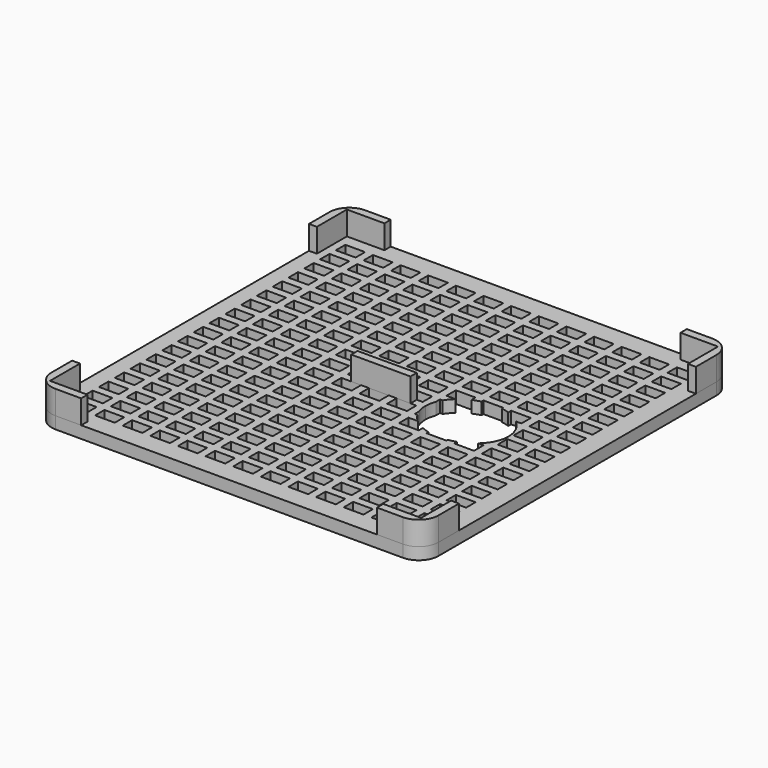
from build123d import *

# Parameters (mm, degrees)
F0_W     = 5
F0_H     = 3
F1_DEPTH = 3.048
F3_DEPTH = 4
F4_W     = 15
F4_H     = 2
F4_W_2   = 2
F4_W_3   = 9.6
F4_H_2   = 9.5
F4_W_4   = 9.5
F5_DEPTH = 6
F6_R     = 5


with BuildPart() as f1:
    # F0 (on Top) → F1 (new body)
    with BuildSketch(Plane.XY):
        Polygon((-42.5, 49), (-49, 49), (-49, 42.5), (-45, 42.5), (-45, 44), (-42.5, 44), align=None)
        Polygon((49, 49), (-42.5, 49), (-42.5, 44), (-40, 44), (-40, 41), (-45, 41), (-45, 42.5), (-49, 42.5), (-49, -49), (49, -49), align=None)
        with Locations((-42.5, -42.5)):
            Rectangle(F0_W, F0_H, mode=Mode.SUBTRACT)
        with Locations((-42.5, -37.5)):
            Rectangle(F0_W, F0_H, mode=Mode.SUBTRACT)
        with Locations((-35.5, -42.5)):
            Rectangle(F0_W, F0_H, mode=Mode.SUBTRACT)
        with Locations((-35.5, -37.5)):
            Rectangle(F0_W, F0_H, mode=Mode.SUBTRACT)
        with Locations((-28.5, -42.5)):
            Rectangle(F0_W, F0_H, mode=Mode.SUBTRACT)
        with Locations((-28.5, -37.5)):
            Rectangle(F0_W, F0_H, mode=Mode.SUBTRACT)
        with Locations((-42.5, -32.5)):
            Rectangle(F0_W, F0_H, mode=Mode.SUBTRACT)
        with Locations((-42.5, -27.5)):
            Rectangle(F0_W, F0_H, mode=Mode.SUBTRACT)
        with Locations((-35.5, -32.5)):
            Rectangle(F0_W, F0_H, mode=Mode.SUBTRACT)
        with Locations((-28.5, -32.5)):
            Rectangle(F0_W, F0_H, mode=Mode.SUBTRACT)
        with Locations((-35.5, -27.5)):
            Rectangle(F0_W, F0_H, mode=Mode.SUBTRACT)
        with Locations((-28.5, -27.5)):
            Rectangle(F0_W, F0_H, mode=Mode.SUBTRACT)
        with Locations((-21.5, -42.5)):
            Rectangle(F0_W, F0_H, mode=Mode.SUBTRACT)
        with Locations((-21.5, -37.5)):
            Rectangle(F0_W, F0_H, mode=Mode.SUBTRACT)
        with Locations((-14.5, -42.5)):
            Rectangle(F0_W, F0_H, mode=Mode.SUBTRACT)
        with Locations((-14.5, -37.5)):
            Rectangle(F0_W, F0_H, mode=Mode.SUBTRACT)
        with Locations((-7.5, -42.5)):
            Rectangle(F0_W, F0_H, mode=Mode.SUBTRACT)
        with Locations((-7.5, -37.5)):
            Rectangle(F0_W, F0_H, mode=Mode.SUBTRACT)
        with Locations((-0.5, -42.5)):
            Rectangle(F0_W, F0_H, mode=Mode.SUBTRACT)
        with Locations((-0.5, -37.5)):
            Rectangle(F0_W, F0_H, mode=Mode.SUBTRACT)
        with Locations((-21.5, -32.5)):
            Rectangle(F0_W, F0_H, mode=Mode.SUBTRACT)
        with Locations((-14.5, -32.5)):
            Rectangle(F0_W, F0_H, mode=Mode.SUBTRACT)
        with Locations((-21.5, -27.5)):
            Rectangle(F0_W, F0_H, mode=Mode.SUBTRACT)
        with Locations((-14.5, -27.5)):
            Rectangle(F0_W, F0_H, mode=Mode.SUBTRACT)
        with Locations((-7.5, -32.5)):
            Rectangle(F0_W, F0_H, mode=Mode.SUBTRACT)
        with Locations((-0.5, -32.5)):
            Rectangle(F0_W, F0_H, mode=Mode.SUBTRACT)
        with Locations((-7.5, -27.5)):
            Rectangle(F0_W, F0_H, mode=Mode.SUBTRACT)
        with Locations((-0.5, -27.5)):
            Rectangle(F0_W, F0_H, mode=Mode.SUBTRACT)
        with Locations((-42.5, -22.5)):
            Rectangle(F0_W, F0_H, mode=Mode.SUBTRACT)
        with Locations((-42.5, -17.5)):
            Rectangle(F0_W, F0_H, mode=Mode.SUBTRACT)
        with Locations((-42.5, -12.5)):
            Rectangle(F0_W, F0_H, mode=Mode.SUBTRACT)
        with Locations((-35.5, -22.5)):
            Rectangle(F0_W, F0_H, mode=Mode.SUBTRACT)
        with Locations((-28.5, -22.5)):
            Rectangle(F0_W, F0_H, mode=Mode.SUBTRACT)
        with Locations((-35.5, -17.5)):
            Rectangle(F0_W, F0_H, mode=Mode.SUBTRACT)
        with Locations((-35.5, -12.5)):
            Rectangle(F0_W, F0_H, mode=Mode.SUBTRACT)
        with Locations((-28.5, -17.5)):
            Rectangle(F0_W, F0_H, mode=Mode.SUBTRACT)
        with Locations((-28.5, -12.5)):
            Rectangle(F0_W, F0_H, mode=Mode.SUBTRACT)
        with Locations((-42.5, -7.5)):
            Rectangle(F0_W, F0_H, mode=Mode.SUBTRACT)
        with Locations((-42.5, -2.5)):
            Rectangle(F0_W, F0_H, mode=Mode.SUBTRACT)
        with Locations((-35.5, -7.5)):
            Rectangle(F0_W, F0_H, mode=Mode.SUBTRACT)
        with Locations((-28.5, -7.5)):
            Rectangle(F0_W, F0_H, mode=Mode.SUBTRACT)
        with Locations((-35.5, -2.5)):
            Rectangle(F0_W, F0_H, mode=Mode.SUBTRACT)
        with Locations((-28.5, -2.5)):
            Rectangle(F0_W, F0_H, mode=Mode.SUBTRACT)
        with Locations((-21.5, -22.5)):
            Rectangle(F0_W, F0_H, mode=Mode.SUBTRACT)
        with Locations((-14.5, -22.5)):
            Rectangle(F0_W, F0_H, mode=Mode.SUBTRACT)
        with Locations((-21.5, -17.5)):
            Rectangle(F0_W, F0_H, mode=Mode.SUBTRACT)
        with Locations((-21.5, -12.5)):
            Rectangle(F0_W, F0_H, mode=Mode.SUBTRACT)
        with Locations((-14.5, -17.5)):
            Rectangle(F0_W, F0_H, mode=Mode.SUBTRACT)
        with Locations((-14.5, -12.5)):
            Rectangle(F0_W, F0_H, mode=Mode.SUBTRACT)
        with Locations((-7.5, -22.5)):
            Rectangle(F0_W, F0_H, mode=Mode.SUBTRACT)
        with Locations((-0.5, -22.5)):
            Rectangle(F0_W, F0_H, mode=Mode.SUBTRACT)
        with Locations((-7.5, -17.5)):
            Rectangle(F0_W, F0_H, mode=Mode.SUBTRACT)
        with Locations((-7.5, -12.5)):
            Rectangle(F0_W, F0_H, mode=Mode.SUBTRACT)
        with Locations((-0.5, -17.5)):
            Rectangle(F0_W, F0_H, mode=Mode.SUBTRACT)
        with Locations((-0.5, -12.5)):
            Rectangle(F0_W, F0_H, mode=Mode.SUBTRACT)
        with Locations((-21.5, -7.5)):
            Rectangle(F0_W, F0_H, mode=Mode.SUBTRACT)
        with Locations((-14.5, -7.5)):
            Rectangle(F0_W, F0_H, mode=Mode.SUBTRACT)
        with Locations((-21.5, -2.5)):
            Rectangle(F0_W, F0_H, mode=Mode.SUBTRACT)
        with Locations((-14.5, -2.5)):
            Rectangle(F0_W, F0_H, mode=Mode.SUBTRACT)
        with Locations((-7.5, -7.5)):
            Rectangle(F0_W, F0_H, mode=Mode.SUBTRACT)
        with Locations((-0.5, -7.5)):
            Rectangle(F0_W, F0_H, mode=Mode.SUBTRACT)
        with Locations((-7.5, -2.5)):
            Rectangle(F0_W, F0_H, mode=Mode.SUBTRACT)
        with Locations((-0.5, -2.5)):
            Rectangle(F0_W, F0_H, mode=Mode.SUBTRACT)
        with Locations((6.5, -42.5)):
            Rectangle(F0_W, F0_H, mode=Mode.SUBTRACT)
        with Locations((6.5, -37.5)):
            Rectangle(F0_W, F0_H, mode=Mode.SUBTRACT)
        with Locations((13.5, -42.5)):
            Rectangle(F0_W, F0_H, mode=Mode.SUBTRACT)
        with Locations((13.5, -37.5)):
            Rectangle(F0_W, F0_H, mode=Mode.SUBTRACT)
        with Locations((20.5, -42.5)):
            Rectangle(F0_W, F0_H, mode=Mode.SUBTRACT)
        with Locations((20.5, -37.5)):
            Rectangle(F0_W, F0_H, mode=Mode.SUBTRACT)
        with Locations((6.5, -32.5)):
            Rectangle(F0_W, F0_H, mode=Mode.SUBTRACT)
        with Locations((6.5, -27.5)):
            Rectangle(F0_W, F0_H, mode=Mode.SUBTRACT)
        with Locations((13.5, -32.5)):
            Rectangle(F0_W, F0_H, mode=Mode.SUBTRACT)
        with Locations((20.5, -32.5)):
            Rectangle(F0_W, F0_H, mode=Mode.SUBTRACT)
        with Locations((13.5, -27.5)):
            Rectangle(F0_W, F0_H, mode=Mode.SUBTRACT)
        with Locations((20.5, -27.5)):
            Rectangle(F0_W, F0_H, mode=Mode.SUBTRACT)
        with Locations((27.5, -42.5)):
            Rectangle(F0_W, F0_H, mode=Mode.SUBTRACT)
        with Locations((27.5, -37.5)):
            Rectangle(F0_W, F0_H, mode=Mode.SUBTRACT)
        with Locations((34.5, -42.5)):
            Rectangle(F0_W, F0_H, mode=Mode.SUBTRACT)
        with Locations((34.5, -37.5)):
            Rectangle(F0_W, F0_H, mode=Mode.SUBTRACT)
        with Locations((41.5, -42.5)):
            Rectangle(F0_W, F0_H, mode=Mode.SUBTRACT)
        with Locations((41.5, -37.5)):
            Rectangle(F0_W, F0_H, mode=Mode.SUBTRACT)
        with Locations((27.5, -32.5)):
            Rectangle(F0_W, F0_H, mode=Mode.SUBTRACT)
        with Locations((34.5, -32.5)):
            Rectangle(F0_W, F0_H, mode=Mode.SUBTRACT)
        with Locations((27.5, -27.5)):
            Rectangle(F0_W, F0_H, mode=Mode.SUBTRACT)
        with Locations((34.5, -27.5)):
            Rectangle(F0_W, F0_H, mode=Mode.SUBTRACT)
        with Locations((41.5, -32.5)):
            Rectangle(F0_W, F0_H, mode=Mode.SUBTRACT)
        with Locations((41.5, -27.5)):
            Rectangle(F0_W, F0_H, mode=Mode.SUBTRACT)
        with Locations((6.5, -22.5)):
            Rectangle(F0_W, F0_H, mode=Mode.SUBTRACT)
        with Locations((6.5, -17.5)):
            Rectangle(F0_W, F0_H, mode=Mode.SUBTRACT)
        with Locations((6.5, -12.5)):
            Rectangle(F0_W, F0_H, mode=Mode.SUBTRACT)
        with Locations((13.5, -22.5)):
            Rectangle(F0_W, F0_H, mode=Mode.SUBTRACT)
        with Locations((20.5, -22.5)):
            Rectangle(F0_W, F0_H, mode=Mode.SUBTRACT)
        with Locations((13.5, -17.5)):
            Rectangle(F0_W, F0_H, mode=Mode.SUBTRACT)
        with Locations((13.5, -12.5)):
            Rectangle(F0_W, F0_H, mode=Mode.SUBTRACT)
        with Locations((20.5, -17.5)):
            Rectangle(F0_W, F0_H, mode=Mode.SUBTRACT)
        with Locations((20.5, -12.5)):
            Rectangle(F0_W, F0_H, mode=Mode.SUBTRACT)
        with Locations((6.5, -7.5)):
            Rectangle(F0_W, F0_H, mode=Mode.SUBTRACT)
        with Locations((6.5, -2.5)):
            Rectangle(F0_W, F0_H, mode=Mode.SUBTRACT)
        with Locations((13.5, -7.5)):
            Rectangle(F0_W, F0_H, mode=Mode.SUBTRACT)
        with Locations((20.5, -7.5)):
            Rectangle(F0_W, F0_H, mode=Mode.SUBTRACT)
        with Locations((13.5, -2.5)):
            Rectangle(F0_W, F0_H, mode=Mode.SUBTRACT)
        with Locations((20.5, -2.5)):
            Rectangle(F0_W, F0_H, mode=Mode.SUBTRACT)
        with Locations((27.5, -22.5)):
            Rectangle(F0_W, F0_H, mode=Mode.SUBTRACT)
        with Locations((34.5, -22.5)):
            Rectangle(F0_W, F0_H, mode=Mode.SUBTRACT)
        with Locations((27.5, -17.5)):
            Rectangle(F0_W, F0_H, mode=Mode.SUBTRACT)
        with Locations((27.5, -12.5)):
            Rectangle(F0_W, F0_H, mode=Mode.SUBTRACT)
        with Locations((34.5, -17.5)):
            Rectangle(F0_W, F0_H, mode=Mode.SUBTRACT)
        with Locations((34.5, -12.5)):
            Rectangle(F0_W, F0_H, mode=Mode.SUBTRACT)
        with Locations((41.5, -22.5)):
            Rectangle(F0_W, F0_H, mode=Mode.SUBTRACT)
        with Locations((41.5, -17.5)):
            Rectangle(F0_W, F0_H, mode=Mode.SUBTRACT)
        with Locations((41.5, -12.5)):
            Rectangle(F0_W, F0_H, mode=Mode.SUBTRACT)
        with Locations((27.5, -7.5)):
            Rectangle(F0_W, F0_H, mode=Mode.SUBTRACT)
        with Locations((34.5, -7.5)):
            Rectangle(F0_W, F0_H, mode=Mode.SUBTRACT)
        with Locations((27.5, -2.5)):
            Rectangle(F0_W, F0_H, mode=Mode.SUBTRACT)
        with Locations((34.5, -2.5)):
            Rectangle(F0_W, F0_H, mode=Mode.SUBTRACT)
        with Locations((41.5, -7.5)):
            Rectangle(F0_W, F0_H, mode=Mode.SUBTRACT)
        with Locations((41.5, -2.5)):
            Rectangle(F0_W, F0_H, mode=Mode.SUBTRACT)
        with Locations((-42.5, 2.5)):
            Rectangle(F0_W, F0_H, mode=Mode.SUBTRACT)
        with Locations((-42.5, 7.5)):
            Rectangle(F0_W, F0_H, mode=Mode.SUBTRACT)
        with Locations((-35.5, 2.5)):
            Rectangle(F0_W, F0_H, mode=Mode.SUBTRACT)
        with Locations((-28.5, 2.5)):
            Rectangle(F0_W, F0_H, mode=Mode.SUBTRACT)
        with Locations((-35.5, 7.5)):
            Rectangle(F0_W, F0_H, mode=Mode.SUBTRACT)
        with Locations((-28.5, 7.5)):
            Rectangle(F0_W, F0_H, mode=Mode.SUBTRACT)
        with Locations((-42.5, 12.5)):
            Rectangle(F0_W, F0_H, mode=Mode.SUBTRACT)
        with Locations((-42.5, 17.5)):
            Rectangle(F0_W, F0_H, mode=Mode.SUBTRACT)
        with Locations((-42.5, 22.5)):
            Rectangle(F0_W, F0_H, mode=Mode.SUBTRACT)
        with Locations((-35.5, 12.5)):
            Rectangle(F0_W, F0_H, mode=Mode.SUBTRACT)
        with Locations((-35.5, 17.5)):
            Rectangle(F0_W, F0_H, mode=Mode.SUBTRACT)
        with Locations((-28.5, 12.5)):
            Rectangle(F0_W, F0_H, mode=Mode.SUBTRACT)
        with Locations((-28.5, 17.5)):
            Rectangle(F0_W, F0_H, mode=Mode.SUBTRACT)
        with Locations((-35.5, 22.5)):
            Rectangle(F0_W, F0_H, mode=Mode.SUBTRACT)
        with Locations((-28.5, 22.5)):
            Rectangle(F0_W, F0_H, mode=Mode.SUBTRACT)
        with Locations((-21.5, 2.5)):
            Rectangle(F0_W, F0_H, mode=Mode.SUBTRACT)
        with Locations((-14.5, 2.5)):
            Rectangle(F0_W, F0_H, mode=Mode.SUBTRACT)
        with Locations((-21.5, 7.5)):
            Rectangle(F0_W, F0_H, mode=Mode.SUBTRACT)
        with Locations((-14.5, 7.5)):
            Rectangle(F0_W, F0_H, mode=Mode.SUBTRACT)
        with Locations((-7.5, 2.5)):
            Rectangle(F0_W, F0_H, mode=Mode.SUBTRACT)
        with Locations((-0.5, 2.5)):
            Rectangle(F0_W, F0_H, mode=Mode.SUBTRACT)
        with Locations((-7.5, 7.5)):
            Rectangle(F0_W, F0_H, mode=Mode.SUBTRACT)
        with Locations((-0.5, 7.5)):
            Rectangle(F0_W, F0_H, mode=Mode.SUBTRACT)
        with Locations((-21.5, 12.5)):
            Rectangle(F0_W, F0_H, mode=Mode.SUBTRACT)
        with Locations((-21.5, 17.5)):
            Rectangle(F0_W, F0_H, mode=Mode.SUBTRACT)
        with Locations((-14.5, 12.5)):
            Rectangle(F0_W, F0_H, mode=Mode.SUBTRACT)
        with Locations((-14.5, 17.5)):
            Rectangle(F0_W, F0_H, mode=Mode.SUBTRACT)
        with Locations((-21.5, 22.5)):
            Rectangle(F0_W, F0_H, mode=Mode.SUBTRACT)
        with Locations((-14.5, 22.5)):
            Rectangle(F0_W, F0_H, mode=Mode.SUBTRACT)
        with Locations((-7.5, 12.5)):
            Rectangle(F0_W, F0_H, mode=Mode.SUBTRACT)
        with Locations((-7.5, 17.5)):
            Rectangle(F0_W, F0_H, mode=Mode.SUBTRACT)
        with Locations((-0.5, 12.5)):
            Rectangle(F0_W, F0_H, mode=Mode.SUBTRACT)
        with Locations((-0.5, 17.5)):
            Rectangle(F0_W, F0_H, mode=Mode.SUBTRACT)
        with Locations((-7.5, 22.5)):
            Rectangle(F0_W, F0_H, mode=Mode.SUBTRACT)
        with Locations((-0.5, 22.5)):
            Rectangle(F0_W, F0_H, mode=Mode.SUBTRACT)
        with Locations((-42.5, 27.5)):
            Rectangle(F0_W, F0_H, mode=Mode.SUBTRACT)
        with Locations((-42.5, 32.5)):
            Rectangle(F0_W, F0_H, mode=Mode.SUBTRACT)
        with Locations((-35.5, 27.5)):
            Rectangle(F0_W, F0_H, mode=Mode.SUBTRACT)
        with Locations((-28.5, 27.5)):
            Rectangle(F0_W, F0_H, mode=Mode.SUBTRACT)
        with Locations((-35.5, 32.5)):
            Rectangle(F0_W, F0_H, mode=Mode.SUBTRACT)
        with Locations((-28.5, 32.5)):
            Rectangle(F0_W, F0_H, mode=Mode.SUBTRACT)
        with Locations((-42.5, 37.5)):
            Rectangle(F0_W, F0_H, mode=Mode.SUBTRACT)
        with Locations((-35.5, 37.5)):
            Rectangle(F0_W, F0_H, mode=Mode.SUBTRACT)
        with Locations((-35.5, 42.5)):
            Rectangle(F0_W, F0_H, mode=Mode.SUBTRACT)
        with Locations((-28.5, 37.5)):
            Rectangle(F0_W, F0_H, mode=Mode.SUBTRACT)
        with Locations((-28.5, 42.5)):
            Rectangle(F0_W, F0_H, mode=Mode.SUBTRACT)
        with Locations((-21.5, 27.5)):
            Rectangle(F0_W, F0_H, mode=Mode.SUBTRACT)
        with Locations((-14.5, 27.5)):
            Rectangle(F0_W, F0_H, mode=Mode.SUBTRACT)
        with Locations((-21.5, 32.5)):
            Rectangle(F0_W, F0_H, mode=Mode.SUBTRACT)
        with Locations((-14.5, 32.5)):
            Rectangle(F0_W, F0_H, mode=Mode.SUBTRACT)
        with Locations((-7.5, 27.5)):
            Rectangle(F0_W, F0_H, mode=Mode.SUBTRACT)
        with Locations((-0.5, 27.5)):
            Rectangle(F0_W, F0_H, mode=Mode.SUBTRACT)
        with Locations((-7.5, 32.5)):
            Rectangle(F0_W, F0_H, mode=Mode.SUBTRACT)
        with Locations((-0.5, 32.5)):
            Rectangle(F0_W, F0_H, mode=Mode.SUBTRACT)
        with Locations((-21.5, 37.5)):
            Rectangle(F0_W, F0_H, mode=Mode.SUBTRACT)
        with Locations((-21.5, 42.5)):
            Rectangle(F0_W, F0_H, mode=Mode.SUBTRACT)
        with Locations((-14.5, 37.5)):
            Rectangle(F0_W, F0_H, mode=Mode.SUBTRACT)
        with Locations((-14.5, 42.5)):
            Rectangle(F0_W, F0_H, mode=Mode.SUBTRACT)
        with Locations((-7.5, 37.5)):
            Rectangle(F0_W, F0_H, mode=Mode.SUBTRACT)
        with Locations((-7.5, 42.5)):
            Rectangle(F0_W, F0_H, mode=Mode.SUBTRACT)
        with Locations((-0.5, 37.5)):
            Rectangle(F0_W, F0_H, mode=Mode.SUBTRACT)
        with Locations((-0.5, 42.5)):
            Rectangle(F0_W, F0_H, mode=Mode.SUBTRACT)
        with Locations((6.5, 2.5)):
            Rectangle(F0_W, F0_H, mode=Mode.SUBTRACT)
        with Locations((6.5, 7.5)):
            Rectangle(F0_W, F0_H, mode=Mode.SUBTRACT)
        with Locations((13.5, 2.5)):
            Rectangle(F0_W, F0_H, mode=Mode.SUBTRACT)
        with Locations((20.5, 2.5)):
            Rectangle(F0_W, F0_H, mode=Mode.SUBTRACT)
        with Locations((13.5, 7.5)):
            Rectangle(F0_W, F0_H, mode=Mode.SUBTRACT)
        with Locations((20.5, 7.5)):
            Rectangle(F0_W, F0_H, mode=Mode.SUBTRACT)
        with Locations((6.5, 12.5)):
            Rectangle(F0_W, F0_H, mode=Mode.SUBTRACT)
        with Locations((6.5, 17.5)):
            Rectangle(F0_W, F0_H, mode=Mode.SUBTRACT)
        with Locations((6.5, 22.5)):
            Rectangle(F0_W, F0_H, mode=Mode.SUBTRACT)
        with Locations((13.5, 12.5)):
            Rectangle(F0_W, F0_H, mode=Mode.SUBTRACT)
        with Locations((13.5, 17.5)):
            Rectangle(F0_W, F0_H, mode=Mode.SUBTRACT)
        with Locations((20.5, 12.5)):
            Rectangle(F0_W, F0_H, mode=Mode.SUBTRACT)
        with Locations((20.5, 17.5)):
            Rectangle(F0_W, F0_H, mode=Mode.SUBTRACT)
        with Locations((13.5, 22.5)):
            Rectangle(F0_W, F0_H, mode=Mode.SUBTRACT)
        with Locations((20.5, 22.5)):
            Rectangle(F0_W, F0_H, mode=Mode.SUBTRACT)
        with Locations((27.5, 2.5)):
            Rectangle(F0_W, F0_H, mode=Mode.SUBTRACT)
        with Locations((34.5, 2.5)):
            Rectangle(F0_W, F0_H, mode=Mode.SUBTRACT)
        with Locations((27.5, 7.5)):
            Rectangle(F0_W, F0_H, mode=Mode.SUBTRACT)
        with Locations((34.5, 7.5)):
            Rectangle(F0_W, F0_H, mode=Mode.SUBTRACT)
        with Locations((41.5, 2.5)):
            Rectangle(F0_W, F0_H, mode=Mode.SUBTRACT)
        with Locations((41.5, 7.5)):
            Rectangle(F0_W, F0_H, mode=Mode.SUBTRACT)
        with Locations((27.5, 12.5)):
            Rectangle(F0_W, F0_H, mode=Mode.SUBTRACT)
        with Locations((27.5, 17.5)):
            Rectangle(F0_W, F0_H, mode=Mode.SUBTRACT)
        with Locations((34.5, 12.5)):
            Rectangle(F0_W, F0_H, mode=Mode.SUBTRACT)
        with Locations((34.5, 17.5)):
            Rectangle(F0_W, F0_H, mode=Mode.SUBTRACT)
        with Locations((27.5, 22.5)):
            Rectangle(F0_W, F0_H, mode=Mode.SUBTRACT)
        with Locations((34.5, 22.5)):
            Rectangle(F0_W, F0_H, mode=Mode.SUBTRACT)
        with Locations((41.5, 12.5)):
            Rectangle(F0_W, F0_H, mode=Mode.SUBTRACT)
        with Locations((41.5, 17.5)):
            Rectangle(F0_W, F0_H, mode=Mode.SUBTRACT)
        with Locations((41.5, 22.5)):
            Rectangle(F0_W, F0_H, mode=Mode.SUBTRACT)
        with Locations((6.5, 27.5)):
            Rectangle(F0_W, F0_H, mode=Mode.SUBTRACT)
        with Locations((6.5, 32.5)):
            Rectangle(F0_W, F0_H, mode=Mode.SUBTRACT)
        with Locations((13.5, 27.5)):
            Rectangle(F0_W, F0_H, mode=Mode.SUBTRACT)
        with Locations((20.5, 27.5)):
            Rectangle(F0_W, F0_H, mode=Mode.SUBTRACT)
        with Locations((13.5, 32.5)):
            Rectangle(F0_W, F0_H, mode=Mode.SUBTRACT)
        with Locations((20.5, 32.5)):
            Rectangle(F0_W, F0_H, mode=Mode.SUBTRACT)
        with Locations((6.5, 37.5)):
            Rectangle(F0_W, F0_H, mode=Mode.SUBTRACT)
        with Locations((6.5, 42.5)):
            Rectangle(F0_W, F0_H, mode=Mode.SUBTRACT)
        with Locations((13.5, 37.5)):
            Rectangle(F0_W, F0_H, mode=Mode.SUBTRACT)
        with Locations((13.5, 42.5)):
            Rectangle(F0_W, F0_H, mode=Mode.SUBTRACT)
        with Locations((20.5, 37.5)):
            Rectangle(F0_W, F0_H, mode=Mode.SUBTRACT)
        with Locations((20.5, 42.5)):
            Rectangle(F0_W, F0_H, mode=Mode.SUBTRACT)
        with Locations((27.5, 27.5)):
            Rectangle(F0_W, F0_H, mode=Mode.SUBTRACT)
        with Locations((34.5, 27.5)):
            Rectangle(F0_W, F0_H, mode=Mode.SUBTRACT)
        with Locations((27.5, 32.5)):
            Rectangle(F0_W, F0_H, mode=Mode.SUBTRACT)
        with Locations((34.5, 32.5)):
            Rectangle(F0_W, F0_H, mode=Mode.SUBTRACT)
        with Locations((41.5, 27.5)):
            Rectangle(F0_W, F0_H, mode=Mode.SUBTRACT)
        with Locations((41.5, 32.5)):
            Rectangle(F0_W, F0_H, mode=Mode.SUBTRACT)
        with Locations((27.5, 37.5)):
            Rectangle(F0_W, F0_H, mode=Mode.SUBTRACT)
        with Locations((27.5, 42.5)):
            Rectangle(F0_W, F0_H, mode=Mode.SUBTRACT)
        with Locations((34.5, 37.5)):
            Rectangle(F0_W, F0_H, mode=Mode.SUBTRACT)
        with Locations((34.5, 42.5)):
            Rectangle(F0_W, F0_H, mode=Mode.SUBTRACT)
        with Locations((41.5, 37.5)):
            Rectangle(F0_W, F0_H, mode=Mode.SUBTRACT)
        with Locations((41.5, 42.5)):
            Rectangle(F0_W, F0_H, mode=Mode.SUBTRACT)
    extrude(amount=F1_DEPTH)

    # F2 (on Top) → F3 (cut)
    with BuildSketch(Plane.XY):
        with BuildLine():
            add(Edge.make_bspline(
                [(10.5, 0), (10.5, -15.1554445662), (26.25, -7.5777222831), (42, 0), (26.25, 7.5777222831), (10.5, 15.1554445662), (10.5, 0)],
                knots=[0, 0, 0, 2.0943951024, 2.0943951024, 4.1887902048, 4.1887902048, 6.2831853072, 6.2831853072, 6.2831853072], degree=2, weights=[1, 0.5, 1, 0.5, 1, 0.5, 1]))
        make_face()
    extrude(amount=F3_DEPTH, mode=Mode.SUBTRACT)

    # F4 (on face) → F5 (join)
    with BuildSketch(Plane.XY.offset(3.048)):
        Rectangle(F4_W, F4_H)
        with Locations((48, -48)):
            Rectangle(F4_W_2, F4_H)
        with Locations((42.2, -48)):
            Rectangle(F4_W_3, F4_H)
        with Locations((48, -42.25)):
            Rectangle(F4_W_2, F4_H_2)
        with Locations((-48, 48)):
            Rectangle(F4_W_2, F4_H)
        with Locations((-42.25, 48)):
            Rectangle(F4_W_4, F4_H)
        with Locations((-48, 42.25)):
            Rectangle(F4_W_2, F4_H_2)
        with Locations((48, 48)):
            Rectangle(F4_W_2, F4_H)
        with Locations((42.25, 48)):
            Rectangle(F4_W_4, F4_H)
        with Locations((48, 42.25)):
            Rectangle(F4_W_2, F4_H_2)
        with Locations((-48, -48)):
            Rectangle(F4_W_2, F4_H)
        with Locations((-42.25, -48)):
            Rectangle(F4_W_4, F4_H)
        with Locations((-48, -42.25)):
            Rectangle(F4_W_2, F4_H_2)
    extrude(amount=F5_DEPTH)

    # F6
    f6_edges = [f1.edges().sort_by_distance(p)[0] for p in [
        (-49, 49, 1.524),
        (-49, 49, 6.048),
        (49, 49, 1.524),
        (49, 49, 6.048),
        (49, -49, 1.524),
        (49, -49, 6.048),
        (-49, -49, 1.524),
    ]]
    fillet(f6_edges, radius=F6_R)


solid = f1.part
